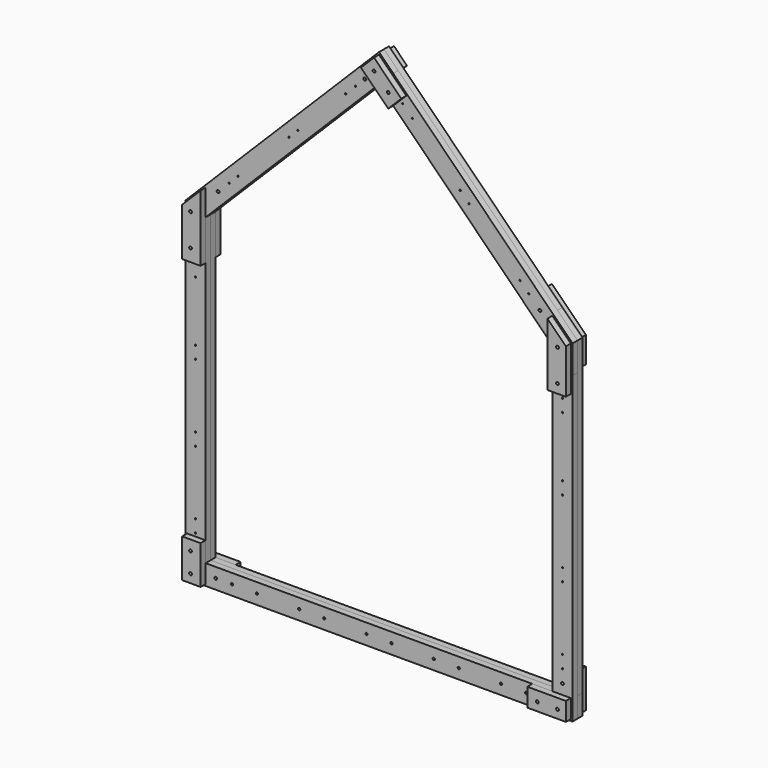
from build123d import *

# Parameters (mm, degrees)
F0_W      = 145
F0_H      = 145
F0_R      = 10
F0_H_2    = 1789.969516728
F1_DEPTH  = 45
F2_DEPTH  = 45
F3_DEPTH  = 45
F4_DEPTH  = 45
F0_W_2    = 2210
F5_DEPTH  = 45
F6_DEPTH  = 45
F7_DEPTH  = 45
F8_DEPTH  = 45
F9_DEPTH  = 45
F10_DEPTH = 45
F11_R     = 10
F12_DEPTH = 45
F11_W     = 133
F11_H     = 145
F11_H_2   = 133
F13_W     = 133
F13_H     = 145
F13_R     = 10
F13_H_2   = 133
F14_DEPTH = 45
F15_DEPTH = 97
F11_R_2   = 5
F11_R_3   = 8
F16_DEPTH = 100


with BuildPart() as f1:
    # F0 (on Front) → F1 (new body)
    with BuildSketch(Plane.XZ):
        with Locations((-4693.0983757973, -2141.7714734616)):
            Rectangle(F0_W, F0_H)
        with Locations((-4693.0983757973, -2141.7714734616)):
            Circle(F0_R, mode=Mode.SUBTRACT)
        with Locations((-4693.0983757973, -1029.2867150977)):
            Rectangle(F0_W, F0_H_2)
        Polygon((-4620.5983757973, -2069.2714734616), (-4620.5983757973, -2024.2714734616), (-4620.5983757973, -1924.2714734616), (-4765.5983757973, -1924.2714734616), (-4765.5983757973, -2069.2714734616), align=None)
        with Locations((-4693.0983757973, -1996.7714734616)):
            Circle(F0_R, mode=Mode.SUBTRACT)
        Polygon((-4620.5983757973, -134.3019567337), (-4620.5983757973, 125.6675599943), (-4765.5983757973, -19.3324400057), (-4765.5983757973, -134.3019567337), align=None)
        with Locations((-4693.0983757973, -74.3019567337)):
            Circle(F0_R, mode=Mode.SUBTRACT)
    extrude(amount=-F1_DEPTH)


with BuildPart() as f2:
    # F0 (on Front) → F2 (new body)
    with BuildSketch(Plane.XZ):
        Polygon((-3473.1288590693, 1273.1370767222), (-3370.5983757973, 1375.6675599943), (-3473.1288590693, 1478.1980432663), (-3575.6593423414, 1375.6675599943), align=None)
        with Locations((-3473.1288590693, 1375.6675599943)):
            Circle(F0_R, mode=Mode.SUBTRACT)
        Polygon((-4436.7721676171, 309.4937681744), (-3473.1288590693, 1273.1370767222), (-3575.6593423414, 1375.6675599943), (-4539.3026508892, 412.0242514464), align=None)
        Polygon((-4620.5983757973, 330.7285265384), (-4620.5983757973, 125.6675599943), (-4436.7721676171, 309.4937681744), (-4539.3026508892, 412.0242514464), align=None)
        with Locations((-4530.4638161244, 318.3326029392)):
            Circle(F0_R, mode=Mode.SUBTRACT)
        Polygon((-4765.5983757973, -19.3324400057), (-4620.5983757973, 125.6675599943), (-4620.5983757973, 330.7285265384), (-4765.5983757973, 185.7285265384), align=None)
        with Locations((-4693.0983757973, 155.6980432663)):
            Circle(F0_R, mode=Mode.SUBTRACT)
    extrude(amount=-F2_DEPTH)


with BuildPart() as f3:
    # F0 (on Front) → F3 (new body)
    with BuildSketch(Plane.XZ):
        Polygon((-3473.1288590693, 1478.1980432663), (-3370.5983757973, 1375.6675599943), (-3268.0678925252, 1478.1980432663), (-3370.5983757973, 1580.7285265384), align=None)
        with Locations((-3370.5983757973, 1478.1980432663)):
            Circle(F0_R, mode=Mode.SUBTRACT)
        Polygon((-3370.5983757973, 1375.6675599943), (-2120.5983757973, 125.6675599943), (-2120.5983757973, 330.7285265384), (-3268.0678925252, 1478.1980432663), align=None)
        with Locations((-2210.7329354702, 318.3326029392)):
            Circle(F0_R, mode=Mode.SUBTRACT)
        with Locations((-3268.0678925252, 1375.6675599943)):
            Circle(F0_R, mode=Mode.SUBTRACT)
    extrude(amount=-F3_DEPTH)


with BuildPart() as f4:
    # F0 (on Front) → F4 (new body)
    with BuildSketch(Plane.XZ):
        Polygon((-2120.5983757973, 330.7285265384), (-2120.5983757973, 125.6675599943), (-1975.5983757973, -19.3324400057), (-1975.5983757973, 185.7285265384), align=None)
        with Locations((-2048.0983757973, 155.6980432663)):
            Circle(F0_R, mode=Mode.SUBTRACT)
        Polygon((-1975.5983757973, -19.3324400057), (-2120.5983757973, 125.6675599943), (-2120.5983757973, -1924.2714734616), (-1975.5983757973, -1924.2714734616), align=None)
        with Locations((-2048.0983757973, -74.3019567337)):
            Circle(F0_R, mode=Mode.SUBTRACT)
        Polygon((-1975.5983757973, -1924.2714734616), (-2120.5983757973, -1924.2714734616), (-2120.5983757973, -2024.2714734616), (-2120.5983757973, -2069.2714734616), (-1975.5983757973, -2069.2714734616), align=None)
        with Locations((-2048.0983757973, -1996.7714734616)):
            Circle(F0_R, mode=Mode.SUBTRACT)
    extrude(amount=-F4_DEPTH)


with BuildPart() as f5:
    # F0 (on Front) → F5 (new body)
    with BuildSketch(Plane.XZ):
        with Locations((-3370.5983757973, -2141.7714734616)):
            Rectangle(F0_W_2, F0_H)
        with Locations((-4548.0983757973, -2141.7714734616)):
            Rectangle(F0_W, F0_H)
        with Locations((-4548.0983757973, -2141.7714734616)):
            Circle(F0_R, mode=Mode.SUBTRACT)
        with Locations((-2193.0983757973, -2141.7714734616)):
            Rectangle(F0_W, F0_H)
        with Locations((-2193.0983757973, -2141.7714734616)):
            Circle(F0_R, mode=Mode.SUBTRACT)
        with Locations((-2048.0983757973, -2141.7714734616)):
            Rectangle(F0_W, F0_H)
        with Locations((-2048.0983757973, -2141.7714734616)):
            Circle(F0_R, mode=Mode.SUBTRACT)
    extrude(amount=-F5_DEPTH)


with BuildPart() as f6:
    # F0 (on Front) → F6 (new body)
    with BuildSketch(Plane.XZ):
        with Locations((-4693.0983757973, -2141.7714734616)):
            Rectangle(F0_W, F0_H)
        with Locations((-4693.0983757973, -2141.7714734616)):
            Circle(F0_R, mode=Mode.SUBTRACT)
        with Locations((-4548.0983757973, -2141.7714734616)):
            Rectangle(F0_W, F0_H)
        with Locations((-4548.0983757973, -2141.7714734616)):
            Circle(F0_R, mode=Mode.SUBTRACT)
        with Locations((-3370.5983757973, -2141.7714734616)):
            Rectangle(F0_W_2, F0_H)
        with Locations((-2193.0983757973, -2141.7714734616)):
            Rectangle(F0_W, F0_H)
        with Locations((-2193.0983757973, -2141.7714734616)):
            Circle(F0_R, mode=Mode.SUBTRACT)
    extrude(amount=F6_DEPTH)


with BuildPart() as f7:
    # F0 (on Front) → F7 (new body)
    with BuildSketch(Plane.XZ):
        Polygon((-4620.5983757973, -2069.2714734616), (-4620.5983757973, -2024.2714734616), (-4620.5983757973, -1924.2714734616), (-4765.5983757973, -1924.2714734616), (-4765.5983757973, -2069.2714734616), align=None)
        with Locations((-4693.0983757973, -1996.7714734616)):
            Circle(F0_R, mode=Mode.SUBTRACT)
        with Locations((-4693.0983757973, -1029.2867150977)):
            Rectangle(F0_W, F0_H_2)
        Polygon((-4620.5983757973, -134.3019567337), (-4620.5983757973, 125.6675599943), (-4765.5983757973, -19.3324400057), (-4765.5983757973, -134.3019567337), align=None)
        with Locations((-4693.0983757973, -74.3019567337)):
            Circle(F0_R, mode=Mode.SUBTRACT)
        Polygon((-4765.5983757973, -19.3324400057), (-4620.5983757973, 125.6675599943), (-4620.5983757973, 330.7285265384), (-4765.5983757973, 185.7285265384), align=None)
        with Locations((-4693.0983757973, 155.6980432663)):
            Circle(F0_R, mode=Mode.SUBTRACT)
    extrude(amount=F7_DEPTH)


with BuildPart() as f8:
    # F0 (on Front) → F8 (new body)
    with BuildSketch(Plane.XZ):
        Polygon((-4620.5983757973, 330.7285265384), (-4620.5983757973, 125.6675599943), (-4436.7721676171, 309.4937681744), (-4539.3026508892, 412.0242514464), align=None)
        with Locations((-4530.4638161244, 318.3326029392)):
            Circle(F0_R, mode=Mode.SUBTRACT)
        Polygon((-4436.7721676171, 309.4937681744), (-3473.1288590693, 1273.1370767222), (-3575.6593423414, 1375.6675599943), (-4539.3026508892, 412.0242514464), align=None)
        Polygon((-3473.1288590693, 1273.1370767222), (-3370.5983757973, 1375.6675599943), (-3473.1288590693, 1478.1980432663), (-3575.6593423414, 1375.6675599943), align=None)
        with Locations((-3473.1288590693, 1375.6675599943)):
            Circle(F0_R, mode=Mode.SUBTRACT)
        Polygon((-3473.1288590693, 1478.1980432663), (-3370.5983757973, 1375.6675599943), (-3268.0678925252, 1478.1980432663), (-3370.5983757973, 1580.7285265384), align=None)
        with Locations((-3370.5983757973, 1478.1980432663)):
            Circle(F0_R, mode=Mode.SUBTRACT)
    extrude(amount=F8_DEPTH)


with BuildPart() as f9:
    # F0 (on Front) → F9 (new body)
    with BuildSketch(Plane.XZ):
        Polygon((-3370.5983757973, 1375.6675599943), (-2120.5983757973, 125.6675599943), (-2120.5983757973, 330.7285265384), (-3268.0678925252, 1478.1980432663), align=None)
        with Locations((-2210.7329354702, 318.3326029392)):
            Circle(F0_R, mode=Mode.SUBTRACT)
        with Locations((-3268.0678925252, 1375.6675599943)):
            Circle(F0_R, mode=Mode.SUBTRACT)
        Polygon((-2120.5983757973, 330.7285265384), (-2120.5983757973, 125.6675599943), (-1975.5983757973, -19.3324400057), (-1975.5983757973, 185.7285265384), align=None)
        with Locations((-2048.0983757973, 155.6980432663)):
            Circle(F0_R, mode=Mode.SUBTRACT)
    extrude(amount=F9_DEPTH)


with BuildPart() as f10:
    # F0 (on Front) → F10 (new body)
    with BuildSketch(Plane.XZ):
        Polygon((-1975.5983757973, -19.3324400057), (-2120.5983757973, 125.6675599943), (-2120.5983757973, -1924.2714734616), (-1975.5983757973, -1924.2714734616), align=None)
        with Locations((-2048.0983757973, -74.3019567337)):
            Circle(F0_R, mode=Mode.SUBTRACT)
        Polygon((-1975.5983757973, -1924.2714734616), (-2120.5983757973, -1924.2714734616), (-2120.5983757973, -2024.2714734616), (-2120.5983757973, -2069.2714734616), (-1975.5983757973, -2069.2714734616), align=None)
        with Locations((-2048.0983757973, -1996.7714734616)):
            Circle(F0_R, mode=Mode.SUBTRACT)
        with Locations((-2048.0983757973, -2141.7714734616)):
            Rectangle(F0_W, F0_H)
        with Locations((-2048.0983757973, -2141.7714734616)):
            Circle(F0_R, mode=Mode.SUBTRACT)
    extrude(amount=F10_DEPTH)


with BuildPart() as f12:
    # F11 (on face) → F12 (new body)
    with BuildSketch(Plane.XZ.offset(45)):
        Polygon((-4753.5983757973, -7.3324400057), (-4753.5983757973, -164.3324400057), (-4620.5983757973, -164.3324400057), (-4620.5983757973, 125.6675599943), align=None)
        with Locations((-4693.0983757973, -74.3019567337)):
            Circle(F11_R, mode=Mode.SUBTRACT)
        Polygon((-4753.5983757973, 180.7579637899), (-4753.5983757973, -7.3324400057), (-4620.5983757973, 125.6675599943), (-4620.5983757973, 313.7579637899), align=None)
        with Locations((-4693.0983757973, 155.6980432663)):
            Circle(F11_R, mode=Mode.SUBTRACT)
    extrude(amount=F12_DEPTH)


with BuildPart() as f12b:
    # F11 (on face) → F12, piece 2 (new body)
    with BuildSketch(Plane.XZ.offset(45)):
        with Locations((-4687.0983757973, -1996.7714734616)):
            Rectangle(F11_W, F11_H)
        with Locations((-4693.0983757973, -1996.7714734616)):
            Circle(F11_R, mode=Mode.SUBTRACT)
        with Locations((-4687.0983757973, -2135.7714734616)):
            Rectangle(F11_W, F11_H_2)
        with Locations((-4693.0983757973, -2141.7714734616)):
            Circle(F11_R, mode=Mode.SUBTRACT)
    extrude(amount=F12_DEPTH)


with BuildPart() as f12c:
    # F11 (on face) → F12, piece 3 (new body)
    with BuildSketch(Plane.XZ.offset(45)):
        Polygon((-2120.5983757973, -2069.2714734616), (-2265.5983757973, -2069.2714734616), (-2265.5983757973, -2202.2714734616), (-1987.5983757973, -2202.2714734616), (-1987.5983757973, -2069.2714734616), align=None)
        with Locations((-2193.0983757973, -2141.7714734616)):
            Circle(F11_R, mode=Mode.SUBTRACT)
        with Locations((-2048.0983757973, -2141.7714734616)):
            Circle(F11_R, mode=Mode.SUBTRACT)
    extrude(amount=F12_DEPTH)


with BuildPart() as f12d:
    # F11 (on face) → F12, piece 4 (new body)
    with BuildSketch(Plane.XZ.offset(45)):
        Polygon((-2120.5983757973, 125.6675599943), (-2120.5983757973, -139.0982121229), (-1987.5983757973, -139.0982121229), (-1987.5983757973, 180.7579637899), (-2120.5983757973, 313.7579637899), align=None)
        with Locations((-2048.0983757973, -74.3019567337)):
            Circle(F11_R, mode=Mode.SUBTRACT)
        with Locations((-2048.0983757973, 155.6980432663)):
            Circle(F11_R, mode=Mode.SUBTRACT)
    extrude(amount=F12_DEPTH)


with BuildPart() as f12e:
    # F11 (on face) → F12, piece 5 (new body)
    with BuildSketch(Plane.XZ.offset(45)):
        Polygon((-3464.6435776951, 1469.7127618921), (-3370.5983757973, 1375.6675599943), (-3268.0678925252, 1273.1370767222), (-3174.0226906274, 1367.18227862), (-3370.5983757973, 1563.7579637899), align=None)
        with Locations((-3370.5983757973, 1478.1980432663)):
            Circle(F11_R, mode=Mode.SUBTRACT)
        with Locations((-3268.0678925252, 1375.6675599943)):
            Circle(F11_R, mode=Mode.SUBTRACT)
    extrude(amount=F12_DEPTH)


with BuildPart() as f14:
    # F13 (on face) → F14 (new body)
    with BuildSketch(Plane(origin=(0, 45, 0), x_dir=(-1, 0, 0), z_dir=(0, 1, 0))):
        with Locations((2054.0983757973, -1996.7714734616)):
            Rectangle(F13_W, F13_H)
        with Locations((2048.0983757973, -1996.7714734616)):
            Circle(F13_R, mode=Mode.SUBTRACT)
        with Locations((2054.0983757973, -2135.7714734616)):
            Rectangle(F13_W, F13_H_2)
    extrude(amount=F14_DEPTH)


with BuildPart() as f14b:
    # F13 (on face) → F14, piece 2 (new body)
    with BuildSketch(Plane(origin=(0, 45, 0), x_dir=(-1, 0, 0), z_dir=(0, 1, 0))):
        Polygon((4620.5983757973, -2069.2714734616), (4475.5983757973, -2069.2714734616), (4475.5983757973, -2202.2714734616), (4765.5983757973, -2202.2714734616), (4765.5983757973, -2069.2714734616), (4753.5983757973, -2069.2714734616), align=None)
    extrude(amount=F14_DEPTH)


with BuildPart() as f14c:
    # F13 (on face) → F14, piece 3 (new body)
    with BuildSketch(Plane(origin=(0, 45, 0), x_dir=(-1, 0, 0), z_dir=(0, 1, 0))):
        Polygon((1987.5983757973, 180.7579637899), (1987.5983757973, -7.3324400057), (2120.5983757973, 125.6675599943), (2120.5983757973, 313.7579637899), align=None)
        with Locations((2048.0983757973, 155.6980432663)):
            Circle(F13_R, mode=Mode.SUBTRACT)
        Polygon((2120.5983757973, 313.7579637899), (2120.5983757973, 125.6675599943), (2325.6593423414, 330.7285265384), (2231.6141404436, 424.7737284362), align=None)
    extrude(amount=F14_DEPTH)


with BuildPart() as f14d:
    # F13 (on face) → F14, piece 4 (new body)
    with BuildSketch(Plane(origin=(0, 45, 0), x_dir=(-1, 0, 0), z_dir=(0, 1, 0))):
        Polygon((4620.5983757973, 125.6675599943), (4620.5983757973, -164.3324400057), (4753.5983757973, -164.3324400057), (4753.5983757973, 180.7579637899), (4620.5983757973, 313.7579637899), align=None)
    extrude(amount=F14_DEPTH)


with BuildPart() as f14e:
    # F13 (on face) → F14, piece 5 (new body)
    with BuildSketch(Plane(origin=(0, 45, 0), x_dir=(-1, 0, 0), z_dir=(0, 1, 0))):
        Polygon((3276.5531738995, 1469.7127618921), (3370.5983757973, 1375.6675599943), (3473.1288590693, 1273.1370767222), (3567.1740609671, 1367.18227862), (3370.5983757973, 1563.7579637899), align=None)
    extrude(amount=F14_DEPTH)


with BuildPart() as f15_tool:
    # F0 (on Front) → F15 (new body)
    with BuildSketch(Plane.XZ):
        with Locations((-3473.1288590693, 1375.6675599943)):
            Circle(F0_R)
        with Locations((-3370.5983757973, 1478.1980432663)):
            Circle(F0_R)
        with Locations((-3268.0678925252, 1375.6675599943)):
            Circle(F0_R)
        with Locations((-4530.4638161244, 318.3326029392)):
            Circle(F0_R)
        with Locations((-4693.0983757973, 155.6980432663)):
            Circle(F0_R)
        with Locations((-4693.0983757973, -74.3019567337)):
            Circle(F0_R)
        with Locations((-4693.0983757973, -1996.7714734616)):
            Circle(F0_R)
        with Locations((-4693.0983757973, -2141.7714734616)):
            Circle(F0_R)
        with Locations((-4548.0983757973, -2141.7714734616)):
            Circle(F0_R)
        with Locations((-2193.0983757973, -2141.7714734616)):
            Circle(F0_R)
        with Locations((-2048.0983757973, -2141.7714734616)):
            Circle(F0_R)
        with Locations((-2048.0983757973, -1996.7714734616)):
            Circle(F0_R)
        with Locations((-2048.0983757973, -74.3019567337)):
            Circle(F0_R)
        with Locations((-2048.0983757973, 155.6980432663)):
            Circle(F0_R)
        with Locations((-2210.7329354702, 318.3326029392)):
            Circle(F0_R)
    extrude(amount=-F15_DEPTH)


with BuildPart() as f14_1:
    add(f14.part)

    # F15: cut by f15_tool
    add(f15_tool.part, mode=Mode.SUBTRACT)


with BuildPart() as f14b_1:
    add(f14b.part)

    # F15: cut by f15_tool
    add(f15_tool.part, mode=Mode.SUBTRACT)


with BuildPart() as f14c_1:
    add(f14c.part)

    # F15: cut by f15_tool
    add(f15_tool.part, mode=Mode.SUBTRACT)


with BuildPart() as f14d_1:
    add(f14d.part)

    # F15: cut by f15_tool
    add(f15_tool.part, mode=Mode.SUBTRACT)


with BuildPart() as f14e_1:
    add(f14e.part)

    # F15: cut by f15_tool
    add(f15_tool.part, mode=Mode.SUBTRACT)


with BuildPart() as f16_tool:
    # F11 (on face) → F16 (new body)
    with BuildSketch(Plane.XZ.offset(45)):
        with Locations((-3540.304003282, 1308.4924157815)):
            Circle(F11_R_2)
        with Locations((-3611.0146814007, 1237.7817376629)):
            Circle(F11_R_2)
        with Locations((-3200.8927483125, 1308.4924157815)):
            Circle(F11_R_2)
        with Locations((-3130.1820701938, 1237.7817376629)):
            Circle(F11_R_2)
        with Locations((-3955.9180014819, 892.8784175817)):
            Circle(F11_R_2)
        with Locations((-4019.5576117887, 829.2388072749)):
            Circle(F11_R_2)
        with Locations((-4387.2531380057, 461.5432810579)):
            Circle(F11_R_2)
        with Locations((-4450.8927483125, 397.9036707511)):
            Circle(F11_R_2)
        with Locations((-4693.0983757973, -186.8324400057)):
            Circle(F11_R_2)
        with Locations((-4693.0983757973, -276.8324400057)):
            Circle(F11_R_2)
        with Locations((-4693.0983757973, -709.7714734616)):
            Circle(F11_R_2)
        with Locations((-4693.0983757973, -799.7714734616)):
            Circle(F11_R_2)
        with Locations((-4693.0983757973, -1260.7714734616)):
            Circle(F11_R_2)
        with Locations((-4693.0983757973, -1350.7714734616)):
            Circle(F11_R_2)
        with Locations((-4693.0983757973, -1811.7714734616)):
            Circle(F11_R_2)
        with Locations((-4693.0983757973, -1901.7714734616)):
            Circle(F11_R_2)
        with Locations((-4430.5983757973, -2141.7714734616)):
            Circle(F11_R_3)
        with Locations((-4250.5983757973, -2141.7714734616)):
            Circle(F11_R_3)
        with Locations((-3945.5983757973, -2141.7714734616)):
            Circle(F11_R_3)
        with Locations((-3460.5983757973, -2141.7714734616)):
            Circle(F11_R_3)
        with Locations((-3280.5983757973, -2141.7714734616)):
            Circle(F11_R_3)
        with Locations((-2975.5983757973, -2141.7714734616)):
            Circle(F11_R_3)
        with Locations((-2795.5983757973, -2141.7714734617)):
            Circle(F11_R_3)
        with Locations((-2490.5983757973, -2141.7714734617)):
            Circle(F11_R_3)
        with Locations((-2310.5983757973, -2141.7714734617)):
            Circle(F11_R_3)
        with Locations((-2048.0983757973, -1901.7714734617)):
            Circle(F11_R_2)
        with Locations((-2048.0983757973, -1811.7714734617)):
            Circle(F11_R_2)
        with Locations((-3765.5983757973, -2141.7714734616)):
            Circle(F11_R_3)
        with Locations((-2048.0983757973, -1350.7714734617)):
            Circle(F11_R_2)
        with Locations((-2048.0983757973, -1260.7714734617)):
            Circle(F11_R_2)
        with Locations((-2048.0983757972, -799.7714734617)):
            Circle(F11_R_2)
        with Locations((-2048.0983757972, -709.7714734617)):
            Circle(F11_R_2)
        with Locations((-2048.0983757972, -276.8324400058)):
            Circle(F11_R_2)
        with Locations((-2048.0983757973, -186.8324400057)):
            Circle(F11_R_2)
        with Locations((-2290.304003282, 397.9036707511)):
            Circle(F11_R_2)
        with Locations((-2353.9436135888, 461.5432810579)):
            Circle(F11_R_2)
        with Locations((-2721.6391398058, 829.2388072749)):
            Circle(F11_R_2)
        with Locations((-2785.2787501126, 892.8784175817)):
            Circle(F11_R_2)
    extrude(amount=-F16_DEPTH)


with BuildPart() as f1_1:
    add(f1.part)

    # F16: cut by f16_tool
    add(f16_tool.part, mode=Mode.SUBTRACT)


with BuildPart() as f2_1:
    add(f2.part)

    # F16: cut by f16_tool
    add(f16_tool.part, mode=Mode.SUBTRACT)


with BuildPart() as f3_1:
    add(f3.part)

    # F16: cut by f16_tool
    add(f16_tool.part, mode=Mode.SUBTRACT)


with BuildPart() as f4_1:
    add(f4.part)

    # F16: cut by f16_tool
    add(f16_tool.part, mode=Mode.SUBTRACT)


with BuildPart() as f5_1:
    add(f5.part)

    # F16: cut by f16_tool
    add(f16_tool.part, mode=Mode.SUBTRACT)


with BuildPart() as f6_1:
    add(f6.part)

    # F16: cut by f16_tool
    add(f16_tool.part, mode=Mode.SUBTRACT)


with BuildPart() as f7_1:
    add(f7.part)

    # F16: cut by f16_tool
    add(f16_tool.part, mode=Mode.SUBTRACT)


with BuildPart() as f8_1:
    add(f8.part)

    # F16: cut by f16_tool
    add(f16_tool.part, mode=Mode.SUBTRACT)


with BuildPart() as f9_1:
    add(f9.part)

    # F16: cut by f16_tool
    add(f16_tool.part, mode=Mode.SUBTRACT)


with BuildPart() as f10_1:
    add(f10.part)

    # F16: cut by f16_tool
    add(f16_tool.part, mode=Mode.SUBTRACT)


solid = Compound([f12.part, f12b.part, f12c.part, f12d.part, f12e.part, f14_1.part, f14b_1.part, f14c_1.part, f14d_1.part, f14e_1.part, f1_1.part, f2_1.part, f3_1.part, f4_1.part, f5_1.part, f6_1.part, f7_1.part, f8_1.part, f9_1.part, f10_1.part])
